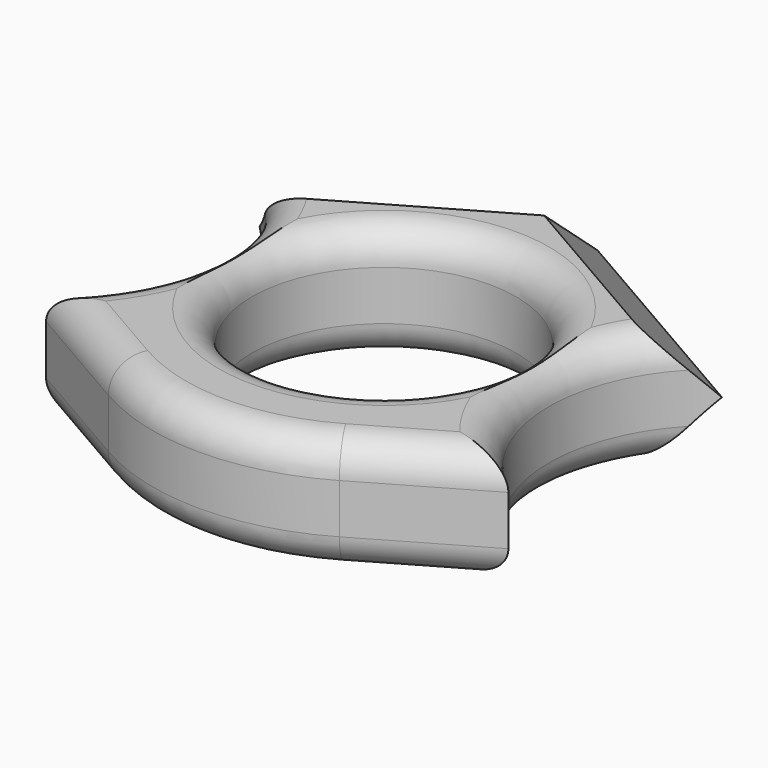
from build123d import *

# Parameters (mm, degrees)
F0_R         = 12.7
F1_DEPTH     = 11.1125
F2_SIZE      = 5.55624
F3_T1_DEPTH  = 20.7691097327
F3_T3_DEPTH  = 20.7691097327
F3_T10_ANGLE = 141.384588939
F3_T12_ANGLE = 141.384588939
F3_T14_ANGLE = 60
F3_T16_ANGLE = 60
F3_T18_ANGLE = 141.384588939
F3_T20_ANGLE = 141.384588939


# Not quite as in the source:
# - a fillet or chamfer that OpenCascade refuses, or shapes differently, is made with other operations: its cross-section is extruded or revolved along the edge and cut away or added
# - a fillet or chamfer is up to 0.001 mm smaller than in the source, because OpenCascade refuses the exact size


with BuildPart() as f1:
    # F0 (on Top) → F1 (new body)
    with BuildSketch(Plane.XY):
        with BuildLine():
            Line((0, 25.6632194655), (-22.225, 12.8316097327))
            ThreePointArc((-22.225, 12.8316097327), (-15.875, 0), (-22.225, -12.8316097327))
            Line((-22.225, -12.8316097327), (-11.1125, -19.2474145991))
            ThreePointArc((-11.1125, -19.2474145991), (0, -22.225), (11.1125, -19.2474145991))
            Line((11.1125, -19.2474145991), (22.225, -12.8316097327))
            ThreePointArc((22.225, -12.8316097327), (15.875, 0), (22.225, 12.8316097327))
            Line((22.225, 12.8316097327), (0, 25.6632194655))
        make_face()
        Circle(F0_R, mode=Mode.SUBTRACT)
    extrude(amount=F1_DEPTH)

    # F2 (size 5.55625 in the source; OpenCascade refuses exactly that, so slightly less here)
    f2_edges = [f1.edges().sort_by_distance(p)[0] for p in [
        (11.1125, 19.247415, 0),
        (11.1125, 19.247415, 11.1125),
        (-11.1125, 19.247415, 11.1125),
        (-11.1125, 19.247415, 0),
    ]]
    chamfer(f2_edges, length=F2_SIZE)

    # F3: fillet of radius 3.175 on 13 edges, made by hand

    # F3_s2 → F3_t1 (cut)
    with BuildSketch(Plane(origin=(-17.9865766425, 10.3845548664, 0), x_dir=(0, 0, 1), z_dir=(0.8660254038, -0.5, 0))):
        with BuildLine():
            ThreePointArc((11.1125, 19.05), (10.1825640303, 21.2950640303), (7.9375, 22.225))
            Line((7.9375, 22.225), (11.1125, 22.225))
            Line((11.1125, 22.225), (11.1125, 19.05))
        make_face()
        with BuildLine():
            ThreePointArc((0, 19.05), (0.9299359697, 21.2950640303), (3.175, 22.225))
            Line((3.175, 22.225), (0, 22.225))
            Line((0, 22.225), (0, 19.05))
        make_face()
    extrude(amount=F3_T1_DEPTH, mode=Mode.SUBTRACT)

    # F3_s4 → F3_t3 (cut)
    with BuildSketch(Plane(origin=(0, 0, 0), x_dir=(0, 0, 1), z_dir=(0.8660254038, 0.5, 0))):
        with BuildLine():
            ThreePointArc((0, 19.05), (0.9299359697, 21.2950640303), (3.175, 22.225))
            Line((3.175, 22.225), (0, 22.225))
            Line((0, 22.225), (0, 19.05))
        make_face()
        with BuildLine():
            ThreePointArc((11.1125, 19.05), (10.1825640303, 21.2950640303), (7.9375, 22.225))
            Line((7.9375, 22.225), (11.1125, 22.225))
            Line((11.1125, 22.225), (11.1125, 19.05))
        make_face()
    extrude(amount=F3_T3_DEPTH, mode=Mode.SUBTRACT)

    # F3_s5 → F3_t6 (revolve, cut)
    with BuildSketch(Plane.XZ):
        with BuildLine():
            ThreePointArc((15.875, 0), (13.6299359697, 0.9299359697), (12.7, 3.175))
            Line((12.7, 3.175), (12.7, 0))
            Line((12.7, 0), (15.875, 0))
        make_face()
    revolve(axis=Axis((0, 0, 0), (0, 0, 1)), mode=Mode.SUBTRACT)

    # F3_s7 → F3_t8 (revolve, cut)
    with BuildSketch(Plane.XZ):
        with BuildLine():
            ThreePointArc((15.875, 11.1125), (13.6299359697, 10.1825640303), (12.7, 7.9375))
            Line((12.7, 7.9375), (12.7, 11.1125))
            Line((12.7, 11.1125), (15.875, 11.1125))
        make_face()
    revolve(axis=Axis((0, 0, 11.1125), (0, 0, 1)), mode=Mode.SUBTRACT)

    # F3_s9 → F3_t10 (revolve, cut)
    with BuildSketch(Plane(origin=(-24.2694814431, 13.7102008228, 0), x_dir=(0, 0, 1), z_dir=(-0.8706754951, 0.4918578882, 0))):
        with BuildLine():
            ThreePointArc((11.1125, 3.567957984), (10.1825640303, 1.3228939538), (7.9375, 0.392957984))
            Line((7.9375, 0.392957984), (11.1125, 0.392957984))
            Line((11.1125, 0.392957984), (11.1125, 3.567957984))
        make_face()
    revolve(axis=Axis((-32.0145833333, 0, 11.1125), (0, 0, -1)), revolution_arc=F3_T10_ANGLE, mode=Mode.SUBTRACT)

    # F3_s11 → F3_t12 (revolve, cut)
    with BuildSketch(Plane(origin=(-24.2694814431, 13.7102008228, 0), x_dir=(0, 0, 1), z_dir=(-0.8706754951, 0.4918578882, 0))):
        with BuildLine():
            ThreePointArc((0, 3.567957984), (0.9299359697, 1.3228939538), (3.175, 0.392957984))
            Line((3.175, 0.392957984), (0, 0.392957984))
            Line((0, 0.392957984), (0, 3.567957984))
        make_face()
    revolve(axis=Axis((-32.0145833333, 0, 0), (0, 0, -1)), revolution_arc=F3_T12_ANGLE, mode=Mode.SUBTRACT)

    # F3_s13 → F3_t14 (revolve, cut)
    with BuildSketch(Plane(origin=(0, 0, 0), x_dir=(0, 0, 1), z_dir=(-0.8660254038, 0.5, 0))):
        with BuildLine():
            ThreePointArc((11.1125, -19.05), (10.1825640303, -21.2950640303), (7.9375, -22.225))
            Line((7.9375, -22.225), (11.1125, -22.225))
            Line((11.1125, -22.225), (11.1125, -19.05))
        make_face()
    revolve(axis=Axis((0, 0, 11.1125), (0, 0, 1)), revolution_arc=F3_T14_ANGLE, mode=Mode.SUBTRACT)

    # F3_s15 → F3_t16 (revolve, cut)
    with BuildSketch(Plane(origin=(0, 0, 0), x_dir=(0, 0, 1), z_dir=(-0.8660254038, 0.5, 0))):
        with BuildLine():
            ThreePointArc((0, -19.05), (0.9299359697, -21.2950640303), (3.175, -22.225))
            Line((3.175, -22.225), (0, -22.225))
            Line((0, -22.225), (0, -19.05))
        make_face()
    revolve(axis=Axis((0, 0, 0), (0, 0, 1)), revolution_arc=F3_T16_ANGLE, mode=Mode.SUBTRACT)

    # F3_s17 → F3_t18 (revolve, cut)
    with BuildSketch(Plane(origin=(31.2045585083, -5.0275706902, 0), x_dir=(0, 0, 1), z_dir=(0.9872680765, -0.1590652226, 0))):
        with BuildLine():
            ThreePointArc((3.175, 11.0471765092), (0.9299359697, 11.977112479), (0, 14.2221765092))
            Line((0, 14.2221765092), (0, 11.0471765092))
            Line((0, 11.0471765092), (3.175, 11.0471765092))
        make_face()
    revolve(axis=Axis((32.0145833333, 0, 0), (0, 0, -1)), revolution_arc=F3_T18_ANGLE, mode=Mode.SUBTRACT)

    # F3_s19 → F3_t20 (revolve, cut)
    with BuildSketch(Plane(origin=(31.2045585083, -5.0275706902, 0), x_dir=(0, 0, 1), z_dir=(0.9872680765, -0.1590652226, 0))):
        with BuildLine():
            ThreePointArc((7.9375, 11.0471765092), (10.1825640303, 11.977112479), (11.1125, 14.2221765092))
            Line((11.1125, 14.2221765092), (11.1125, 11.0471765092))
            Line((11.1125, 11.0471765092), (7.9375, 11.0471765092))
        make_face()
    revolve(axis=Axis((32.0145833333, 0, 11.1125), (0, 0, -1)), revolution_arc=F3_T20_ANGLE, mode=Mode.SUBTRACT)


solid = f1.part
